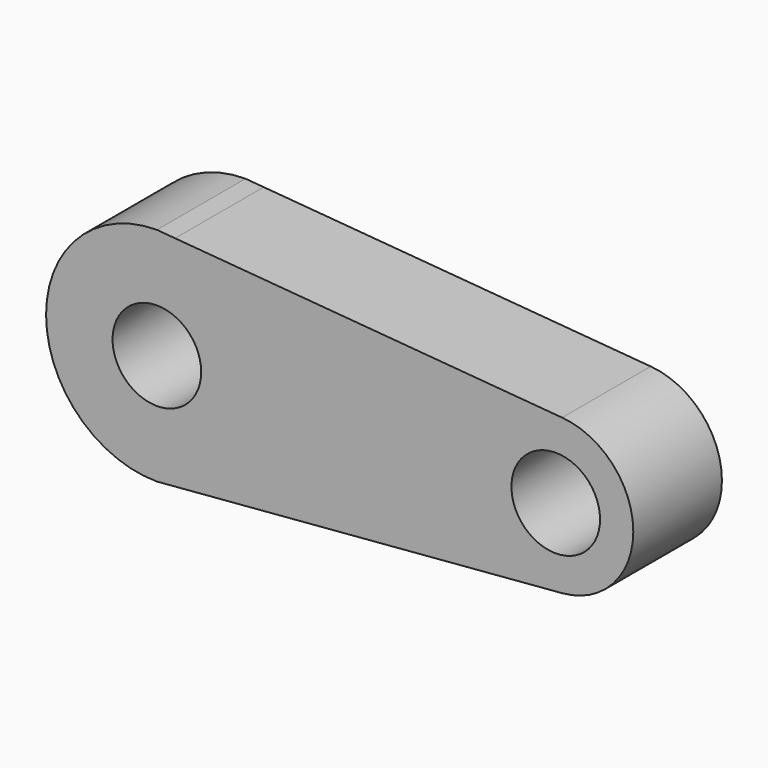
from build123d import *

# Parameters (mm, degrees)
F0_R     = 10
F1_DEPTH = 25


with BuildPart() as f1:
    # F0 (on Front) → F1 (new body)
    with BuildSketch(Plane.XZ):
        with BuildLine():
            Line((4.1054428346, 24.6606029758), (0, 25))
            ThreePointArc((0, 25), (-25, 0), (0, -25))
            Line((0, -25), (4.1054428346, -24.6606029758))
            ThreePointArc((4.1054428346, -24.6606029758), (19.0740146648, -16.1611251022), (25, 0))
            ThreePointArc((25, 0), (19.0740146648, 16.1611251022), (4.1054428346, 24.6606029758))
        make_face()
        Circle(F0_R, mode=Mode.SUBTRACT)
        with BuildLine():
            Line((91.4418067738, 17.4405043857), (4.1054428346, 24.6606029758))
            ThreePointArc((4.1054428346, 24.6606029758), (19.0740146648, 16.1611251022), (25, 0))
            ThreePointArc((25, 0), (19.0740146648, -16.1611251022), (4.1054428346, -24.6606029758))
            Line((4.1054428346, -24.6606029758), (91.4418067738, -17.4405043857))
            ThreePointArc((91.4418067738, -17.4405043857), (72.5, 0), (91.4418067738, 17.4405043857))
        make_face()
        with BuildLine():
            ThreePointArc((107.5, 0), (102.8740362463, 11.8536572723), (91.4418067738, 17.4405043857))
            ThreePointArc((91.4418067738, 17.4405043857), (72.5, 0), (91.4418067738, -17.4405043857))
            ThreePointArc((91.4418067738, -17.4405043857), (102.8740362463, -11.8536572723), (107.5, 0))
        make_face()
        with Locations((90, 0)):
            Circle(F0_R, mode=Mode.SUBTRACT)
    extrude(amount=F1_DEPTH)


solid = f1.part
